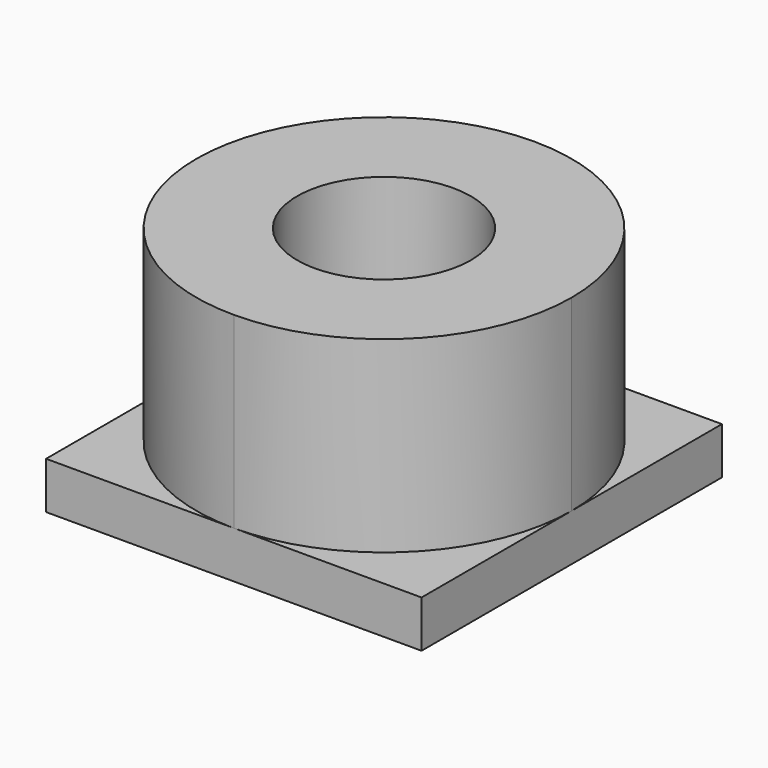
from build123d import *

# Parameters (mm, degrees)
F0_R     = 1.85
F1_DEPTH = 1
F2_DEPTH = 5


with BuildPart() as f1:
    # F0 (on Top) → F1 (new body)
    with BuildSketch(Plane.XY):
        with BuildLine():
            ThreePointArc((4, 0), (2.8284271247, 2.8284271247), (0, 4))
            ThreePointArc((0, 4), (-2.8284271247, 2.8284271247), (-4, 0))
            ThreePointArc((-4, 0), (-2.8284271247, -2.8284271247), (0, -4))
            ThreePointArc((0, -4), (2.8284271247, -2.8284271247), (4, 0))
        make_face()
        Circle(F0_R, mode=Mode.SUBTRACT)
        with BuildLine():
            Line((0, 4), (-4, 4))
            Line((-4, 4), (-4, 0))
            ThreePointArc((-4, 0), (-2.8284271247, 2.8284271247), (0, 4))
        make_face()
        with BuildLine():
            Line((4, 4), (0, 4))
            ThreePointArc((0, 4), (2.8284271247, 2.8284271247), (4, 0))
            Line((4, 0), (4, 4))
        make_face()
        with BuildLine():
            ThreePointArc((0, -4), (-2.8284271247, -2.8284271247), (-4, 0))
            Line((-4, 0), (-4, -4))
            Line((-4, -4), (0, -4))
        make_face()
        with BuildLine():
            Line((4, -4), (4, 0))
            ThreePointArc((4, 0), (2.8284271247, -2.8284271247), (0, -4))
            Line((0, -4), (4, -4))
        make_face()
    extrude(amount=F1_DEPTH)

    # F0 (on Top) → F2 (join)
    with BuildSketch(Plane.XY):
        with BuildLine():
            ThreePointArc((4, 0), (2.8284271247, 2.8284271247), (0, 4))
            ThreePointArc((0, 4), (-2.8284271247, 2.8284271247), (-4, 0))
            ThreePointArc((-4, 0), (-2.8284271247, -2.8284271247), (0, -4))
            ThreePointArc((0, -4), (2.8284271247, -2.8284271247), (4, 0))
        make_face()
        Circle(F0_R, mode=Mode.SUBTRACT)
    extrude(amount=F2_DEPTH)


solid = f1.part
